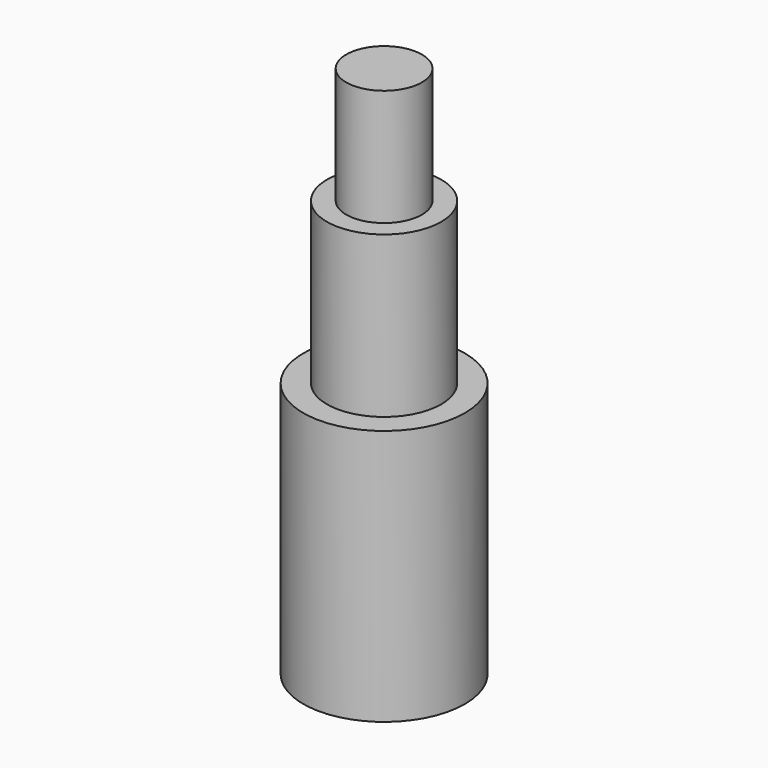
from build123d import *

# Parameters (mm, degrees)
F0_R     = 14.9949916
F0_R_2   = 10.5999915
F1_DEPTH = 47.50999896
F0_R_3   = 7.01499994
F2_DEPTH = 98.9000054
F3_DEPTH = 77.301598


with BuildPart() as f1:
    # F0 (on Top) → F1 (new body)
    with BuildSketch(Plane.XY):
        Circle(F0_R)
        Circle(F0_R_2, mode=Mode.SUBTRACT)
    extrude(amount=F1_DEPTH)

    # F0 (on Top) → F3 (join)
    with BuildSketch(Plane.XY):
        Circle(F0_R_2)
        Circle(F0_R_3, mode=Mode.SUBTRACT)
    extrude(amount=F3_DEPTH)


with BuildPart() as f2:
    # F0 (on Top) → F2 (new body)
    with BuildSketch(Plane.XY):
        Circle(F0_R_3)
    extrude(amount=F2_DEPTH)


solid = Compound([f1.part, f2.part])
